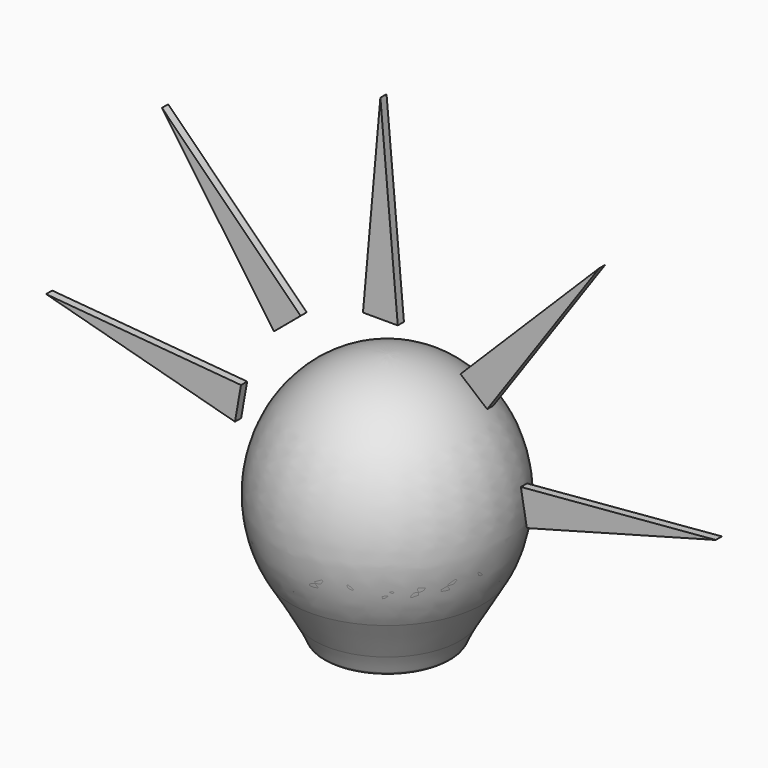
from build123d import *

# Parameters (mm, degrees)
F2_T     = -0.1
F4_DEPTH = 2
F6_COUNT = 3
F6_ANGLE = 80
F7_COUNT = 3
F7_ANGLE = 80


# Not quite as in the source:
# - a shell that OpenCascade refuses in one call is made with other operations: the cavity is built on its own and cut out


with BuildPart() as f1:
    # F0 (on Front) → F1 (revolve)
    with BuildSketch(Plane.XZ):
        with BuildLine():
            Line((-15.4683816494, 0), (0, 0))
            Line((0, 0), (0, 65))
            add(Edge.make_bspline(
                [(0, 65), (-53.6115006556, 65), (-24.9198123266, 15.8303619511)],
                knots=[0, 0, 0, 2.135514613, 2.135514613, 2.135514613], degree=2, weights=[1, 0.4820903118, 1]))
            Line((-24.9198123266, 15.8303619511), (-18.8718817936, 5.4658775806))
            ThreePointArc((-18.8718817936, 5.4658775806), (-17.6054522133, 3.1172637552), (-16.5, 0.6887238263))
            ThreePointArc((-16.5, 0.6887238263), (-16.0885785799, 0.188002688), (-15.4683816494, 0))
        make_face()
    revolve(axis=Axis((0, 0, 32.5), (0, 0, 1)))

    # F2: a shell. OpenCascade refuses it in one call, so the cavity is built on its own and cut out:
    # the body offset inwards by the wall thickness, plus a prism from it out through each open face.
    f2_core = offset(f1.part, amount=F2_T, mode=Mode.PRIVATE)
    f2_exits = [f2_core.faces().sort_by_distance(p)[0] for p in [
        (0, 0, 0.1),
    ]]
    add(f2_core, mode=Mode.SUBTRACT)
    extrude(f2_exits, amount=-F2_T, mode=Mode.SUBTRACT)


with BuildPart() as f4:
    # F3 (on Front) → F4 (new body)
    with BuildSketch(Plane.XZ):
        Polygon((4.3439801882, 73.6905180782), (-0.1720996806, 124.2893819253), (-4.6881795495, 73.6905180782), align=None)
    extrude(amount=F4_DEPTH)


with BuildPart() as f6_1:
    # F6: instance of F4
    add(f4.part.rotate(Axis((0, 0, 36), (0, 1, 0)), 1 * F6_ANGLE / (F6_COUNT - 1)))


with BuildPart() as f6_2:
    # F6: instance of F4
    add(f4.part.rotate(Axis((0, 0, 36), (0, 1, 0)), 2 * F6_ANGLE / (F6_COUNT - 1)))


with BuildPart() as f7_1:
    # F7: instance of F4
    add(f4.part.rotate(Axis((0, 0, 36), (0, -1, 0)), 1 * F7_ANGLE / (F7_COUNT - 1)))


with BuildPart() as f7_2:
    # F7: instance of F4
    add(f4.part.rotate(Axis((0, 0, 36), (0, -1, 0)), 2 * F7_ANGLE / (F7_COUNT - 1)))


solid = Compound([f1.part, f4.part, f6_1.part, f6_2.part, f7_1.part, f7_2.part])
